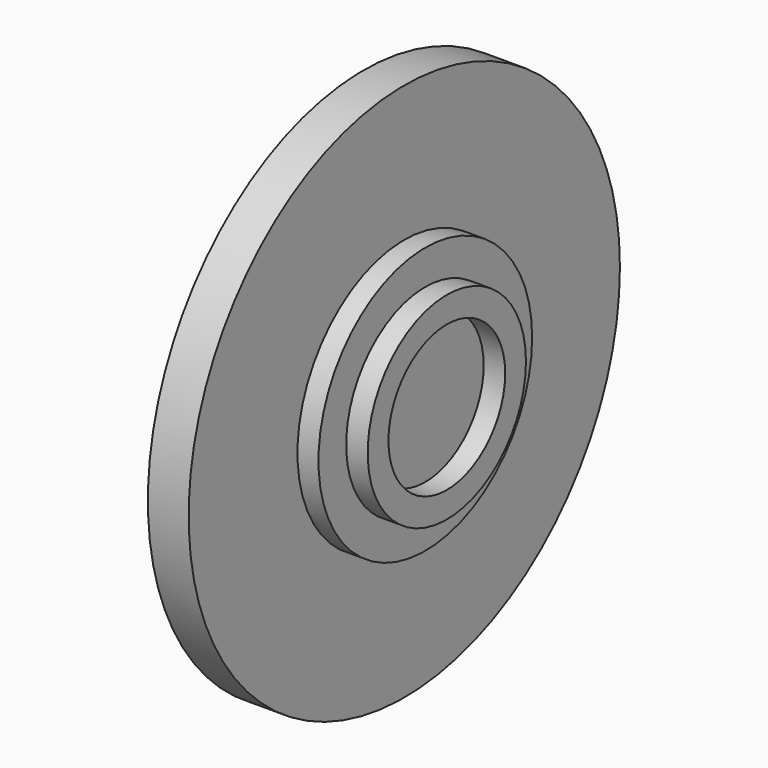
from build123d import *

# Parameters (mm, degrees)
F0_R      = 10.9
F1_DEPTH  = 1.65
F2_R      = 4
F3_DEPTH  = 3.37
F5_R      = 2.95
F6_DEPTH  = 3.37
F7_R      = 2.98
F8_DEPTH  = 1.65
F9_R      = 5.4
F10_DEPTH = 2.5


# Not quite as in the source:
# - a feature names something its author has since deleted; it is built from what else it names


with BuildPart() as f1:
    # F0 (on Right) → F1 (new body)
    with BuildSketch(Plane.YZ):
        Circle(F0_R)
    extrude(amount=F1_DEPTH)

    # F2 (on Right) → F3 (join)
    with BuildSketch(Plane.YZ):
        Circle(F2_R)
    extrude(amount=F3_DEPTH)

    # F5 (on offset) → F6 (cut)
    with BuildSketch(Plane.YZ.offset(3.37)):
        Circle(F5_R)
    extrude(amount=-F6_DEPTH, mode=Mode.SUBTRACT)

    # F7 (on Right) → F8 (join)
    with BuildSketch(Plane.YZ):
        Circle(F7_R)
    extrude(amount=F8_DEPTH)

    # F9 (on Right) → F10 (join)
    with BuildSketch(Plane.YZ):
        Circle(F9_R)
    extrude(amount=F10_DEPTH)


solid = f1.part
